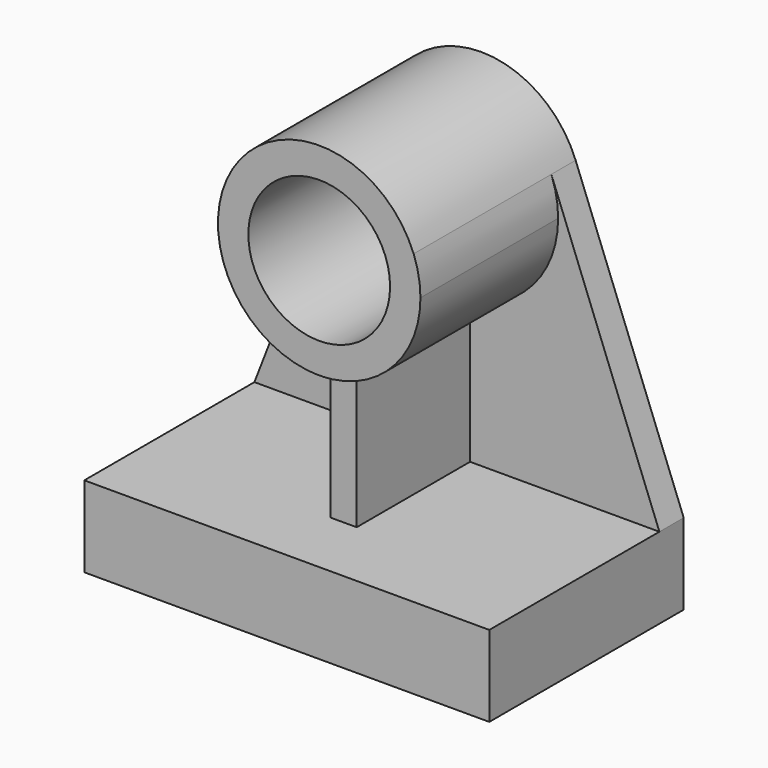
from build123d import *

# Parameters (mm, degrees)
F2_DEPTH = 107.95
F3_DEPTH = 19.05
F4_DEPTH = 19.05
F1_R     = 44.45
F5_DEPTH = 127
F6_DEPTH = 152.4


# Not quite as in the source:
# - a variable given as a bare number and used for a length is read in inches; the dataset says mm whatever the document's units were


with BuildPart() as f2:
    # F1 (on Front) → F2 (new body)
    with BuildSketch(Plane.XZ):
        with BuildLine():
            Line((118.745, 140.2388613905), (118.745, 50.8))
            Line((118.745, 50.8), (135.255, 50.8))
            Line((135.255, 50.8), (135.255, 140.2388613905))
            ThreePointArc((135.255, 140.2388613905), (127, 139.7), (118.745, 140.2388613905))
        make_face()
    extrude(amount=F2_DEPTH)

    # F1 (on Front) → F3 (join)
    with BuildSketch(Plane.XZ):
        with BuildLine():
            Line((135.255, 50.8), (254, 50.8))
            Line((254, 50.8), (186.2277468166, 226.0981223472))
            ThreePointArc((186.2277468166, 226.0981223472), (189.4228000127, 214.8466320699), (190.5, 203.2))
            ThreePointArc((190.5, 203.2), (174.7307160013, 161.3188735825), (135.255, 140.2388613905))
            Line((135.255, 140.2388613905), (135.255, 50.8))
        make_face()
    extrude(amount=F3_DEPTH)

    # F1 (on Front) → F4 (join)
    with BuildSketch(Plane.XZ):
        with BuildLine():
            Line((67.7722531834, 226.0981223472), (0, 50.8))
            Line((0, 50.8), (118.745, 50.8))
            Line((118.745, 50.8), (118.745, 140.2388613905))
            ThreePointArc((118.745, 140.2388613905), (72.3974959138, 170.7836993549), (67.7722531834, 226.0981223472))
        make_face()
    extrude(amount=F4_DEPTH)

    # F1 (on Front) → F5 (join)
    with BuildSketch(Plane.XZ):
        with BuildLine():
            ThreePointArc((186.2277468166, 226.0981223472), (127, 266.7), (67.7722531834, 226.0981223472))
            ThreePointArc((67.7722531834, 226.0981223472), (72.3974959138, 170.7836993549), (118.745, 140.2388613905))
            ThreePointArc((118.745, 140.2388613905), (127, 139.7), (135.255, 140.2388613905))
            ThreePointArc((135.255, 140.2388613905), (174.7307160013, 161.3188735825), (190.5, 203.2))
            ThreePointArc((190.5, 203.2), (189.4228000127, 214.8466320699), (186.2277468166, 226.0981223472))
        make_face()
        with Locations((127, 203.2)):
            Circle(F1_R, mode=Mode.SUBTRACT)
    extrude(amount=F5_DEPTH)

    # F1 (on Front) → F6 (join)
    with BuildSketch(Plane.XZ):
        Polygon((0, 50.8), (0, 0), (254, 0), (254, 50.8), (135.255, 50.8), (118.745, 50.8), align=None)
    extrude(amount=F6_DEPTH)


solid = f2.part
